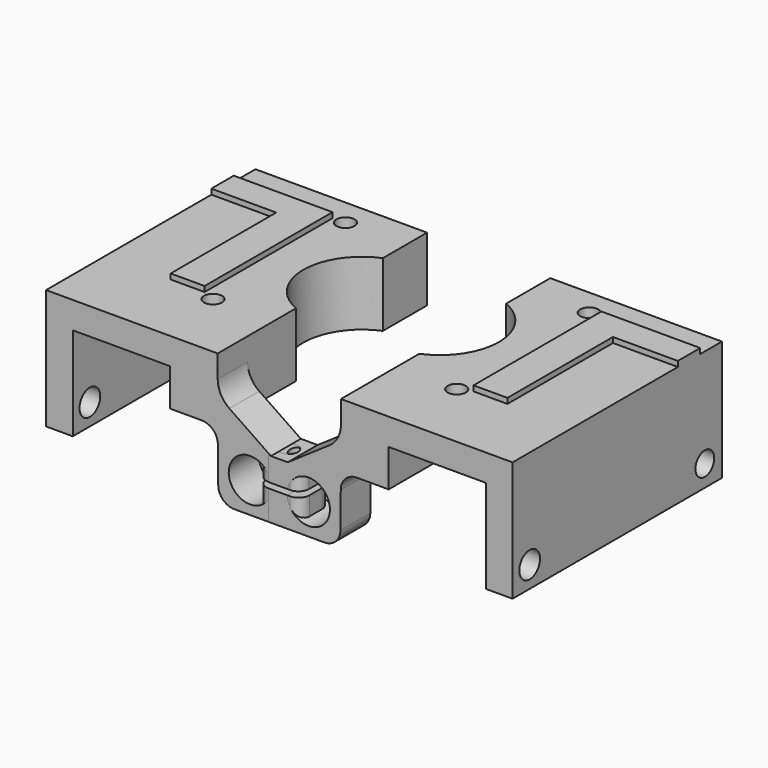
from build123d import *

# Parameters (mm, degrees)
F1_DEPTH      = 7
F2_DEPTH      = 42
F3_R          = 1.7
F3_R_2        = 11
F4_DEPTH      = 12.001
F5_R          = 4
F6_DEPTH      = 10
F7_DEPTH      = 12.001
F8_R          = 1.4
F9_DEPTH      = 10.9920075553
F8_R_2        = 1.7
F10_DEPTH     = 4.4348209087
F11_R         = 5
F12_R         = 3
F13_R         = 3
F14_R         = 2
F15_R         = 2.2
F15_R_2       = 2.4255023423
F16_DEPTH     = 6
F17_TEXT_SIZE = 41.9437823343
F18_DEPTH     = 1


# Not quite as in the source:
# - a feature names something its author has since deleted; it is built from what else it names
# - Text() gives the source's letters only with a copy of the font that has no kerning and outlines rounded to 1/6400 em; it was checked with that copy


with BuildPart() as f1:
    # F0 (on Front) → F1 (new body)
    with BuildSketch(Plane.XZ):
        Polygon((-18.6721007523, 29.8099789735), (-18.6721007523, 7.3259699669), (-13.6721007523, 7.3259699669), (-13.6721007523, 24.8099789735), (4.5278992477, 24.8099789735), (4.5278992477, 17.8099789735), (13.4637966118, 17.8099789735), (13.4637966118, 22.9406704692), (13.4637966118, 29.8099789735), align=None)
        Polygon((23.4301751077, 16.1394868046), (13.4637966118, 22.9406704692), (13.4637966118, 17.8099789735), (13.5940201178, 5.1484792493), (29.0186601057, 5.1484792493), (29.0186601057, 10.6682249423), (21.6860510706, 10.6682249423), (21.6860510706, 11.7046658959), (28.9896428882, 11.7046658959), (28.9896428882, 16.1394868046), align=None)
    extrude(amount=F1_DEPTH)

    # F0 (on Front) → F2 (join)
    with BuildSketch(Plane.XZ):
        Polygon((-18.6721007523, 29.8099789735), (-18.6721007523, 7.3259699669), (-13.6721007523, 7.3259699669), (-13.6721007523, 24.8099789735), (4.5278992477, 24.8099789735), (4.5278992477, 17.8099789735), (13.4637966118, 17.8099789735), (13.4637966118, 22.9406704692), (13.4637966118, 29.8099789735), align=None)
    extrude(amount=-F2_DEPTH)

    # F3 (on face) → F4 (cut, through all)
    with BuildSketch(Plane(origin=(0, 0, 17.8099789735), x_dir=(1, 0, 0), z_dir=(0, 0, -1))):
        with Locations((2.1850741468, -6)):
            Circle(F3_R)
        with Locations((2.1850741468, -37)):
            Circle(F3_R)
        with Locations((17.6850741468, -21.5)):
            Circle(F3_R_2)
    extrude(amount=-F4_DEPTH, mode=Mode.SUBTRACT)

    # F5 (on face) → F6 (cut)
    with BuildSketch(Plane.XZ.offset(7)):
        with Locations((19.5278992477, 10.8989789735)):
            Circle(F5_R)
    extrude(amount=-F6_DEPTH, mode=Mode.SUBTRACT)

    # F3 (on face) → F7 (cut, through all)
    with BuildSketch(Plane(origin=(0, 0, 17.8099789735), x_dir=(1, 0, 0), z_dir=(0, 0, -1))):
        with Locations((2.1850741468, -6)):
            Circle(F3_R)
        with Locations((2.1850741468, -37)):
            Circle(F3_R)
        with Locations((17.6850741468, -21.5)):
            Circle(F3_R_2)
    extrude(amount=-F7_DEPTH, mode=Mode.SUBTRACT)

    # F8 (on face) → F9 (cut, through all)
    with BuildSketch(Plane.XY.offset(16.1394868046)):
        with Locations((25.9896428882, -3.5767070949)):
            Circle(F8_R)
    extrude(amount=-F9_DEPTH, mode=Mode.SUBTRACT)

    # F8 (on face) → F10 (cut, through all)
    with BuildSketch(Plane.XY.offset(16.1394868046)):
        with Locations((25.9896428882, -3.5767070949)):
            Circle(F8_R_2)
        with Locations((25.9896428882, -3.5767070949)):
            Circle(F8_R, mode=Mode.SUBTRACT)
    extrude(amount=-F10_DEPTH, mode=Mode.SUBTRACT)

    # F11
    f11_edges = [f1.edges().sort_by_distance(p)[0] for p in [
        (13.463797, -3.5, 22.94067),
    ]]
    fillet(f11_edges, radius=F11_R)

    # F12
    f12_edges = [f1.edges().sort_by_distance(p)[0] for p in [
        (13.463797, -3.5, 17.809979),
    ]]
    fillet(f12_edges, radius=F12_R)

    # F13
    f13_edges = [f1.edges().sort_by_distance(p)[0] for p in [
        (13.59402, -3.5, 5.148479),
    ]]
    fillet(f13_edges, radius=F13_R)

    # F14
    f14_edges = [f1.edges().sort_by_distance(p)[0] for p in [
        (28.989643, -7, 13.922076),
        (29.01866, -7, 7.908352),
        (28.989643, 0, 13.922076),
        (29.01866, 0, 7.908352),
    ]]
    fillet(f14_edges, radius=F14_R)

    # F15 (on face) → F16 (cut)
    with BuildSketch(Plane(origin=(-18.6721007523, 0, 0), x_dir=(0, -1, 0), z_dir=(-1, 0, 0))):
        with Locations((-38, 11.3259699669)):
            Circle(F15_R)
        with Locations((3, 11.3259699669)):
            Circle(F15_R_2)
    extrude(amount=-F16_DEPTH, mode=Mode.SUBTRACT)

    # F17 (on face) → F18 (join)
    with BuildSketch(Plane.XY.offset(29.8099789735)):
        with Locations(Location((3.5908724648, 36.9253193088), (0, 0, 180))):
            Text('L', F17_TEXT_SIZE, font='Open Sans', font_style=FontStyle.BOLD, text_align=(TextAlign.LEFT, TextAlign.BOTTOM))
    extrude(amount=F18_DEPTH)


with BuildPart() as f19_1:
    # F19: instance of F1
    add(f1.part.mirror(Plane.YZ))


with BuildPart() as f19_1_1:
    # F20: moved
    add(f19_1.part.moved(Location((50, 0, 0))))


solid = Compound([f1.part, f19_1_1.part])
